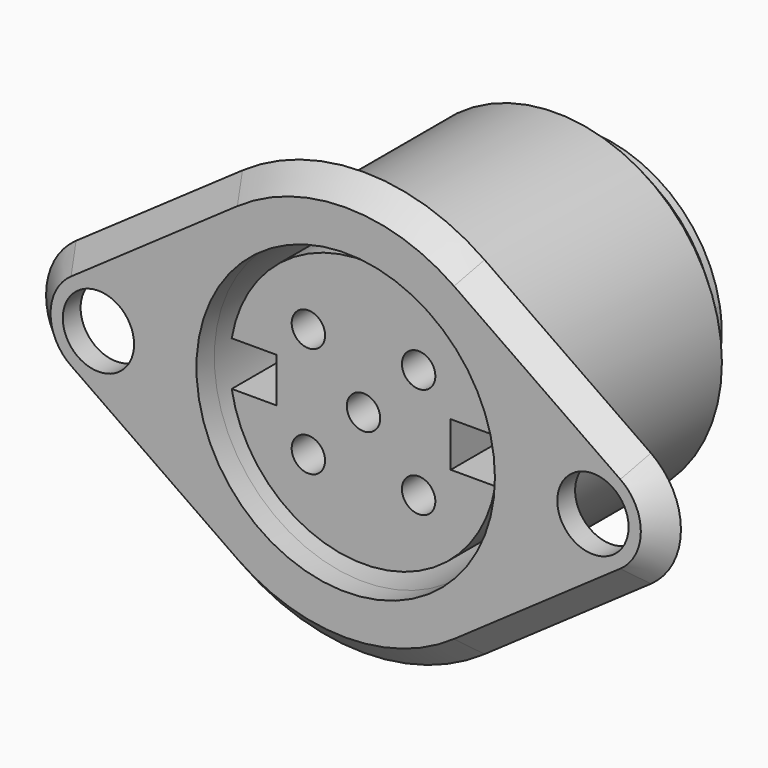
from build123d import *

# Parameters (mm, degrees)
F0_R     = 1.6
F0_R_2   = 7.45
F0_R_3   = 6.7
F1_DEPTH = 1
F2_SIZE  = 0.99999
F0_R_4   = 0.75
F3_DEPTH = 12.1
F4_T     = 0.75
F5_DEPTH = 12.6
F6_DEPTH = 10
F7_SIZE  = 1.3


# Not quite as in the source:
# - a fillet or chamfer is up to 0.001 mm smaller than in the source, because OpenCascade refuses the exact size
# - a shell that OpenCascade refuses in one call is made with other operations: the cavity is built on its own and cut out
# - a feature names something its author has since deleted; it is built from what else it names


with BuildPart() as f1:
    # F0 (on Front) → F1 (new body)
    with BuildSketch(Plane.XZ):
        with BuildLine():
            Line((-5.4346846847, 7.7919318771), (-12.902027027, 2.5836405698))
            ThreePointArc((-12.902027027, 2.5836405698), (-14.25, 0), (-12.902027027, -2.5836405698))
            Line((-12.902027027, -2.5836405698), (-5.4346846847, -7.7919318771))
            ThreePointArc((-5.4346846847, -7.7919318771), (0, -9.5), (5.4346846847, -7.7919318771))
            Line((5.4346846847, -7.7919318771), (12.902027027, -2.5836405698))
            ThreePointArc((12.902027027, -2.5836405698), (14.25, 0), (12.902027027, 2.5836405698))
            Line((12.902027027, 2.5836405698), (5.4346846847, 7.7919318771))
            ThreePointArc((5.4346846847, 7.7919318771), (0, 9.5), (-5.4346846847, 7.7919318771))
        make_face()
        with Locations((-11.1, 0)):
            Circle(F0_R, mode=Mode.SUBTRACT)
        Circle(F0_R_2, mode=Mode.SUBTRACT)
        with Locations((11.1, 0)):
            Circle(F0_R, mode=Mode.SUBTRACT)
        Circle(F0_R_2)
        Circle(F0_R_3, mode=Mode.SUBTRACT)
    extrude(amount=F1_DEPTH)

    # F2 (size 1 in the source; OpenCascade refuses exactly that, so slightly less here)
    f2_edges = [f1.edges().sort_by_distance(p)[0] for p in [
        (-9.168356, -1, 5.187786),
        (0, -1, 9.5),
        (-14.25, -1, 0),
        (-9.168356, -1, -5.187786),
        (0, -1, -9.5),
        (9.168356, -1, -5.187786),
        (14.25, -1, 0),
        (9.168356, -1, 5.187786),
    ]]
    chamfer(f2_edges, length=F2_SIZE)

    # F0 (on Front) → F3 (join)
    with BuildSketch(Plane.XZ):
        Circle(F0_R_2)
        Circle(F0_R_3, mode=Mode.SUBTRACT)
        Circle(F0_R_3)
        with BuildLine():
            ThreePointArc((5.9160797831, 1), (5.9789831367, 0.5017575617), (6, 0))
            ThreePointArc((6, 0), (5.9789831367, -0.5017575617), (5.9160797831, -1))
            ThreePointArc((5.9160797831, -1), (0, -6), (-5.9160797831, -1))
            ThreePointArc((-5.9160797831, -1), (-6, 0), (-5.9160797831, 1))
            ThreePointArc((-5.9160797831, 1), (0, 6), (5.9160797831, 1))
        make_face(mode=Mode.SUBTRACT)
        with BuildLine():
            Line((3.9160797831, 1), (5.9160797831, 1))
            ThreePointArc((5.9160797831, 1), (0, 6), (-5.9160797831, 1))
            Line((-5.9160797831, 1), (-3.9160797831, 1))
            Line((-3.9160797831, 1), (-3.9160797831, -1))
            Line((-3.9160797831, -1), (-5.9160797831, -1))
            ThreePointArc((-5.9160797831, -1), (0, -6), (5.9160797831, -1))
            Line((5.9160797831, -1), (3.9160797831, -1))
            Line((3.9160797831, -1), (3.9160797831, 1))
        make_face()
        with Locations((-2.4748737342, -2.4748737342)):
            Circle(F0_R_4, mode=Mode.SUBTRACT)
        with Locations((2.4748737342, -2.4748737342)):
            Circle(F0_R_4, mode=Mode.SUBTRACT)
        with Locations((-2.4748737342, 2.4748737342)):
            Circle(F0_R_4, mode=Mode.SUBTRACT)
        Circle(F0_R_4, mode=Mode.SUBTRACT)
        with Locations((2.4748737342, 2.4748737342)):
            Circle(F0_R_4, mode=Mode.SUBTRACT)
        with Locations((-2.4748737342, -2.4748737342)):
            Circle(F0_R_4)
        with Locations((2.4748737342, -2.4748737342)):
            Circle(F0_R_4)
        with Locations((-2.4748737342, 2.4748737342)):
            Circle(F0_R_4)
        with Locations((2.4748737342, 2.4748737342)):
            Circle(F0_R_4)
        with BuildLine():
            Line((-3.9160797831, 1), (-5.9160797831, 1))
            ThreePointArc((-5.9160797831, 1), (-6, 0), (-5.9160797831, -1))
            Line((-5.9160797831, -1), (-3.9160797831, -1))
            Line((-3.9160797831, -1), (-3.9160797831, 1))
        make_face()
        with BuildLine():
            ThreePointArc((5.9160797831, -1), (5.9789831367, -0.5017575617), (6, 0))
            ThreePointArc((6, 0), (5.9789831367, 0.5017575617), (5.9160797831, 1))
            Line((5.9160797831, 1), (3.9160797831, 1))
            Line((3.9160797831, 1), (3.9160797831, -1))
            Line((3.9160797831, -1), (5.9160797831, -1))
        make_face()
        Circle(F0_R_4)
    extrude(amount=-F3_DEPTH)

    # F4: shell of thickness 0.75, made by hand


with BuildPart() as f4_core1:
    # F4_t2: copy of F1
    add(f1.part)

    # the walls: a layer under each face that stays
    f4_faces = [f4_core1.faces().sort_by_distance(p)[0] for p in [
        (0, -5e-06, 9.5),
        (9.1683558559, -5e-06, 5.1877862235),
        (0, -0.500005, 9.000005),
        (-12.2142857143, 0, -2.7142857143),
        (-9.1683558559, -5e-06, 5.1877862235),
        (14.25, -5e-06, 0),
        (8.8823226802, -0.500005, 4.7776886467),
        (-8.83334, -1, 0),
        (-8.8823226802, -0.500005, 4.7776886467),
        (-14.25, -5e-06, 0),
        (9.1683558559, -5e-06, -5.1877862235),
        (-9.1683558559, -5e-06, -5.1877862235),
        (0, -5e-06, -9.5),
        (-12.7, -0.5, 0),
        (-7.45, 6.05, 0),
        (9.5, -0.5, 0),
        (13.750005, -0.500005, 0),
        (-13.750005, -0.500005, 0),
        (-8.8823226802, -0.500005, -4.7776886467),
        (0, -0.500005, -9.000005),
        (8.8823226802, -0.500005, -4.7776886467),
        (-6.7, -0.5, 0),
        (0, 12.1, 0),
    ]]
    thicken(f4_faces, amount=-F4_T, mode=Mode.SUBTRACT)

    # F4_s3 → F4_t4 (revolve, cut)
    with BuildSketch(Plane.XY):
        Polygon((7.4575, 0.0075), (7.45, -0.75), (6.7, -0.75), (6.7, 0), align=None)
    revolve(axis=Axis((0, 0, 0), (0, -1, 0)), mode=Mode.SUBTRACT)


with BuildPart() as f1_1:
    add(f1.part)

    # what is left inside the walls is the cavity
    f4_cavity = [f4_core1.part.solids().sort_by_distance(p)[0] for p in [
        (-6.6925, 7.566667, 0),
    ]]
    add(f4_cavity, mode=Mode.SUBTRACT)

    # F7
    f7_edges = [f1_1.edges().sort_by_distance(p)[0] for p in [
        (-7.45, 12.1, 0),
    ]]
    chamfer(f7_edges, length=F7_SIZE)


with BuildPart() as f5:
    # F0 (on Front) → F5 (new body)
    with BuildSketch(Plane.XZ):
        with BuildLine():
            Line((3.9160797831, 1), (5.9160797831, 1))
            ThreePointArc((5.9160797831, 1), (0, 6), (-5.9160797831, 1))
            Line((-5.9160797831, 1), (-3.9160797831, 1))
            Line((-3.9160797831, 1), (-3.9160797831, -1))
            Line((-3.9160797831, -1), (-5.9160797831, -1))
            ThreePointArc((-5.9160797831, -1), (0, -6), (5.9160797831, -1))
            Line((5.9160797831, -1), (3.9160797831, -1))
            Line((3.9160797831, -1), (3.9160797831, 1))
        make_face()
        with Locations((-2.4748737342, -2.4748737342)):
            Circle(F0_R_4, mode=Mode.SUBTRACT)
        with Locations((2.4748737342, -2.4748737342)):
            Circle(F0_R_4, mode=Mode.SUBTRACT)
        with Locations((-2.4748737342, 2.4748737342)):
            Circle(F0_R_4, mode=Mode.SUBTRACT)
        Circle(F0_R_4, mode=Mode.SUBTRACT)
        with Locations((2.4748737342, 2.4748737342)):
            Circle(F0_R_4, mode=Mode.SUBTRACT)
        with BuildLine():
            Line((-3.9160797831, 1), (-5.9160797831, 1))
            ThreePointArc((-5.9160797831, 1), (-6, 0), (-5.9160797831, -1))
            Line((-5.9160797831, -1), (-3.9160797831, -1))
            Line((-3.9160797831, -1), (-3.9160797831, 1))
        make_face()
        with BuildLine():
            ThreePointArc((5.9160797831, -1), (5.9789831367, -0.5017575617), (6, 0))
            ThreePointArc((6, 0), (5.9789831367, 0.5017575617), (5.9160797831, 1))
            Line((5.9160797831, 1), (3.9160797831, 1))
            Line((3.9160797831, 1), (3.9160797831, -1))
            Line((3.9160797831, -1), (5.9160797831, -1))
        make_face()
        with Locations((-2.4748737342, 2.4748737342)):
            Circle(F0_R_4)
        with Locations((2.4748737342, 2.4748737342)):
            Circle(F0_R_4)
        with Locations((-2.4748737342, -2.4748737342)):
            Circle(F0_R_4)
        with Locations((2.4748737342, -2.4748737342)):
            Circle(F0_R_4)
        Circle(F0_R_4)
    extrude(amount=-F5_DEPTH)

    # F0 (on Front) → F6 (cut)
    with BuildSketch(Plane.XZ):
        with Locations((-2.4748737342, -2.4748737342)):
            Circle(F0_R_4)
        with Locations((-2.4748737342, 2.4748737342)):
            Circle(F0_R_4)
        with Locations((2.4748737342, 2.4748737342)):
            Circle(F0_R_4)
        with Locations((2.4748737342, -2.4748737342)):
            Circle(F0_R_4)
        Circle(F0_R_4)
        with BuildLine():
            Line((-3.9160797831, 1), (-5.9160797831, 1))
            ThreePointArc((-5.9160797831, 1), (-6, 0), (-5.9160797831, -1))
            Line((-5.9160797831, -1), (-3.9160797831, -1))
            Line((-3.9160797831, -1), (-3.9160797831, 1))
        make_face()
        with BuildLine():
            ThreePointArc((5.9160797831, -1), (5.9789831367, -0.5017575617), (6, 0))
            ThreePointArc((6, 0), (5.9789831367, 0.5017575617), (5.9160797831, 1))
            Line((5.9160797831, 1), (3.9160797831, 1))
            Line((3.9160797831, 1), (3.9160797831, -1))
            Line((3.9160797831, -1), (5.9160797831, -1))
        make_face()
    extrude(amount=-F6_DEPTH, mode=Mode.SUBTRACT)


solid = Compound([f1_1.part, f5.part])
